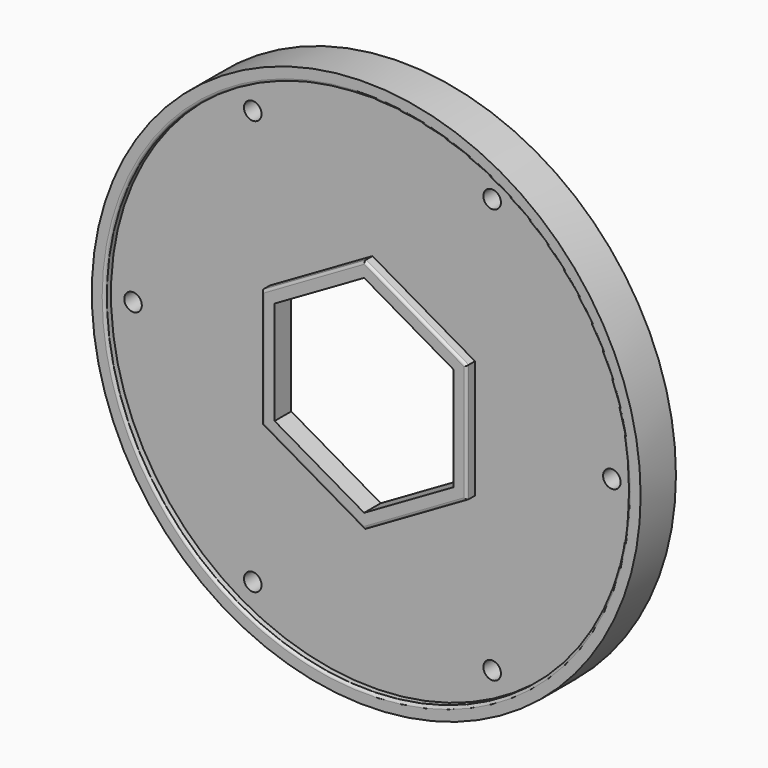
from build123d import *

# Parameters (mm, degrees)
F0_R          = 100.75
F0_R_2        = 5
F0_R_3        = 5.5430968475
F1_DEPTH      = 4
F2_DEPTH      = 4
F3_DEPTH      = 8
F0_R_4        = 105.75
F4_DEPTH      = 7
F6_R          = 1
F7_D          = 6.7564
F8_R          = 1
F9_DEPTH      = 7
F10_DEPTH     = 10
F11_D         = 6.7564
F12_R         = 1
F0_W          = 20
F0_H          = 5
F0_W_2        = 5
F0_H_2        = 20
F13_DEPTH     = 4
F14_DEPTH     = 12
F15_R         = 2
F16_T1_DEPTH  = 8
F16_T3_DEPTH  = 8
F16_T5_DEPTH  = 8
F16_T7_DEPTH  = 8
F16_S11_W     = 2
F16_S11_H     = 2
F16_T12_DEPTH = 2
F16_S17_W     = 2
F16_S17_H     = 2
F16_T18_DEPTH = 2
F16_S23_W     = 2
F16_S23_H     = 2
F16_T24_DEPTH = 2
F16_S29_W     = 2
F16_S29_H     = 2
F16_T30_DEPTH = 2
F16_S35_W     = 2
F16_S35_H     = 2
F16_T36_DEPTH = 2
F16_S41_W     = 2
F16_S41_H     = 2
F16_T42_DEPTH = 2
F16_S47_W     = 2
F16_S47_H     = 2
F16_T48_DEPTH = 2
F16_S53_W     = 2
F16_S53_H     = 2
F16_T54_DEPTH = 2


# Not quite as in the source:
# - a fillet or chamfer that OpenCascade refuses, or shapes differently, is made with other operations: its cross-section is extruded or revolved along the edge and cut away or added
# - a feature names something its author has since deleted; it is built from what else it names


with BuildPart() as f1:
    # F0 (on Front) → F1 (new body)
    with BuildSketch(Plane.XZ):
        Circle(F0_R)
        with Locations((-46.125, -79.8908434991)):
            Circle(F0_R_2, mode=Mode.SUBTRACT)
        with Locations((46.125, -79.8908434991)):
            Circle(F0_R_3, mode=Mode.SUBTRACT)
        with Locations((-92.25, 0)):
            Circle(F0_R_2, mode=Mode.SUBTRACT)
        with Locations((-46.125, 79.8908434991)):
            Circle(F0_R_2, mode=Mode.SUBTRACT)
        Polygon((80.5, 46.4766966698), (80.5, -46.4766966698), (0, -92.9533933395), (-80.5, -46.4766966698), (-80.5, 46.4766966698), (0, 92.9533933395), align=None, mode=Mode.SUBTRACT)
        with Locations((92.25, 0)):
            Circle(F0_R_2, mode=Mode.SUBTRACT)
        with Locations((46.125, 79.8908434991)):
            Circle(F0_R_2, mode=Mode.SUBTRACT)
        with Locations((46.125, 79.8908434991)):
            Circle(F0_R_2)
        with Locations((92.25, 0)):
            Circle(F0_R_2)
        with Locations((46.125, -79.8908434991)):
            Circle(F0_R_3)
        with Locations((-46.125, -79.8908434991)):
            Circle(F0_R_2)
        with Locations((-92.25, 0)):
            Circle(F0_R_2)
        with Locations((-46.125, 79.8908434991)):
            Circle(F0_R_2)
    extrude(amount=F1_DEPTH)



with BuildPart() as f1b:
    # F0 (on Front) → F1, piece 2 (new body)
    with BuildSketch(Plane.XZ):
        Polygon((77.5, -44.7446458622), (77.5, 44.7446458622), (0, 89.4892917244), (-77.5, 44.7446458622), (-77.5, -44.7446458622), (0, -89.4892917244), align=None)
        Polygon((49.9, -10), (49.9, -49.9), (10, -49.9), (10, -54.9), (-10, -54.9), (-10, -49.9), (-49.9, -49.9), (-49.9, -10), (-54.9, -10), (-54.9, 10), (-49.9, 10), (-49.9, 49.9), (-10, 49.9), (-10, 54.9), (10, 54.9), (10, 49.9), (49.9, 49.9), (49.9, 10), (54.9, 10), (54.9, -10), align=None, mode=Mode.SUBTRACT)
        Polygon((10, -49.9), (49.9, -49.9), (49.9, -10), (49.9, 10), (49.9, 49.9), (10, 49.9), (-10, 49.9), (-49.9, 49.9), (-49.9, 10), (-49.9, -10), (-49.9, -49.9), (-10, -49.9), align=None)
        Polygon((39.5, 22.805335633), (39.5, -22.805335633), (0, -45.610671266), (-39.5, -22.805335633), (-39.5, 22.805335633), (0, 45.610671266), align=None, mode=Mode.SUBTRACT)
    extrude(amount=F1_DEPTH)


with BuildPart() as f1_1:
    add(f1.part)

    add(f1b.part)  # F2 merges F1b
    # F0 (on Front) → F2 (join)
    with BuildSketch(Plane.XZ):
        Polygon((0, -92.9533933395), (80.5, -46.4766966698), (80.5, 46.4766966698), (0, 92.9533933395), (-80.5, 46.4766966698), (-80.5, -46.4766966698), align=None)
        Polygon((0, 89.4892917244), (77.5, 44.7446458622), (77.5, -44.7446458622), (0, -89.4892917244), (-77.5, -44.7446458622), (-77.5, 44.7446458622), align=None, mode=Mode.SUBTRACT)
    extrude(amount=F2_DEPTH)

    # F0 (on Front) → F3 (join)
    with BuildSketch(Plane.XZ):
        Polygon((0, -45.610671266), (39.5, -22.805335633), (39.5, 22.805335633), (0, 45.610671266), (-39.5, 22.805335633), (-39.5, -22.805335633), align=None)
        Polygon((34.5, 19.918584287), (34.5, -19.918584287), (0, -39.8371685741), (-34.5, -19.918584287), (-34.5, 19.918584287), (0, 39.8371685741), align=None, mode=Mode.SUBTRACT)
    extrude(amount=F3_DEPTH)

    # F0 (on Front) → F4 (join)
    with BuildSketch(Plane.XZ):
        Circle(F0_R_4)
        Circle(F0_R, mode=Mode.SUBTRACT)
    extrude(amount=F4_DEPTH)

    # F5: union 

    # F6
    f6_edges = [f1_1.edges().sort_by_distance(p)[0] for p in [
        (19.75, -8, 34.208003),
        (39.5, -8, 0),
        (19.75, -8, -34.208003),
        (-19.75, -8, -34.208003),
        (-39.5, -8, 0),
        (-19.75, -8, 34.208003),
    ]]
    fillet(f6_edges, radius=F6_R)

    # F7 (through all)
    with Locations(Plane(origin=(0, 0, 0), x_dir=(1, 0, 0), z_dir=(0, 1, 0))):
        with Locations((-46.125, -79.8908434991), (46.125, -79.8908434991), (92.25, 0), (46.125, 79.8908434991), (-46.125, 79.8908434991), (-92.25, 0)):
            Hole(F7_D / 2)

    # F8
    f8_edges = [f1_1.edges().sort_by_distance(p)[0] for p in [
        (-100.75, -7, 0),
    ]]
    fillet(f8_edges, radius=F8_R)

    # F0 (on Front) → F9 (join)
    with BuildSketch(Plane.XZ):
        with Locations((-46.125, 79.8908434991)):
            Circle(F0_R_2)
        with Locations((46.125, 79.8908434991)):
            Circle(F0_R_2)
        with Locations((92.25, 0)):
            Circle(F0_R_2)
        with Locations((46.125, -79.8908434991)):
            Circle(F0_R_3)
        with Locations((-46.125, -79.8908434991)):
            Circle(F0_R_2)
        with Locations((-92.25, 0)):
            Circle(F0_R_2)
    extrude(amount=-F9_DEPTH)

    # F0 (on Front) → F10 (join)
    with BuildSketch(Plane.XZ):
        Circle(F0_R_4)
        Circle(F0_R, mode=Mode.SUBTRACT)
    extrude(amount=-F10_DEPTH)

    # F11 (through all)
    with Locations(Plane.XZ):
        with Locations((-46.125, 79.8908434991), (46.125, 79.8908434991), (92.25, 0), (46.125, -79.8908434991), (-46.125, -79.8908434991), (-92.25, 0)):
            Hole(F11_D / 2)

    # F12
    f12_edges = [f1_1.edges().sort_by_distance(p)[0] for p in [
        (-100.75, 10, 0),
    ]]
    fillet(f12_edges, radius=F12_R)

    # F0 (on Front) → F13 (join)
    with BuildSketch(Plane.XZ):
        with Locations((0, -52.4)):
            Rectangle(F0_W, F0_H)
        with Locations((52.4, 0)):
            Rectangle(F0_W_2, F0_H_2)
        with Locations((0, 52.4)):
            Rectangle(F0_W, F0_H)
        with Locations((-52.4, 0)):
            Rectangle(F0_W_2, F0_H_2)
    extrude(amount=F13_DEPTH)

    # F0 (on Front) → F14 (join)
    with BuildSketch(Plane.XZ):
        with Locations((0, -52.4)):
            Rectangle(F0_W, F0_H)
        with Locations((52.4, 0)):
            Rectangle(F0_W_2, F0_H_2)
        with Locations((0, 52.4)):
            Rectangle(F0_W, F0_H)
        with Locations((-52.4, 0)):
            Rectangle(F0_W_2, F0_H_2)
    extrude(amount=-F14_DEPTH)

    # F15
    f15_edges = [f1_1.edges().sort_by_distance(p)[0] for p in [
        (0, 12, -49.9),
        (49.9, 12, 0),
        (0, 12, 49.9),
        (-49.9, 12, 0),
        (-10, 6, -49.9),
        (49.9, 6, 10),
        (49.9, 6, -10),
        (10, 6, -49.9),
        (-49.9, 6, -10),
        (-49.9, 6, 10),
        (-10, 6, 49.9),
        (10, 6, 49.9),
    ]]
    fillet(f15_edges, radius=F15_R)

    # F16: fillet of radius 2 on 8 edges, made by hand

    # F16_s2 → F16_t1 (cut)
    with BuildSketch(Plane.XY.offset(-59.9)):
        with BuildLine():
            ThreePointArc((-10, 10), (-9.4142135624, 11.4142135624), (-8, 12))
            Line((-8, 12), (-10, 12))
            Line((-10, 12), (-10, 10))
        make_face()
        with BuildLine():
            ThreePointArc((10, 10), (9.4142135624, 11.4142135624), (8, 12))
            Line((8, 12), (10, 12))
            Line((10, 12), (10, 10))
        make_face()
    extrude(amount=F16_T1_DEPTH, mode=Mode.SUBTRACT)

    # F16_s4 → F16_t3 (cut)
    with BuildSketch(Plane.YZ.offset(51.9)):
        with BuildLine():
            ThreePointArc((10, 10), (11.4142135624, 9.4142135624), (12, 8))
            Line((12, 8), (12, 10))
            Line((12, 10), (10, 10))
        make_face()
        with BuildLine():
            ThreePointArc((10, -10), (11.4142135624, -9.4142135624), (12, -8))
            Line((12, -8), (12, -10))
            Line((12, -10), (10, -10))
        make_face()
    extrude(amount=F16_T3_DEPTH, mode=Mode.SUBTRACT)

    # F16_s6 → F16_t5 (cut)
    with BuildSketch(Plane.XY.offset(51.9)):
        with BuildLine():
            ThreePointArc((10, 10), (9.4142135624, 11.4142135624), (8, 12))
            Line((8, 12), (10, 12))
            Line((10, 12), (10, 10))
        make_face()
        with BuildLine():
            ThreePointArc((-10, 10), (-9.4142135624, 11.4142135624), (-8, 12))
            Line((-8, 12), (-10, 12))
            Line((-10, 12), (-10, 10))
        make_face()
    extrude(amount=F16_T5_DEPTH, mode=Mode.SUBTRACT)

    # F16_s8 → F16_t7 (cut)
    with BuildSketch(Plane.YZ.offset(-59.9)):
        with BuildLine():
            ThreePointArc((10, 10), (11.4142135624, 9.4142135624), (12, 8))
            Line((12, 8), (12, 10))
            Line((12, 10), (10, 10))
        make_face()
        with BuildLine():
            ThreePointArc((10, -10), (11.4142135624, -9.4142135624), (12, -8))
            Line((12, -8), (12, -10))
            Line((12, -10), (10, -10))
        make_face()
    extrude(amount=F16_T7_DEPTH, mode=Mode.SUBTRACT)


with BuildPart() as f16_tool10:
    # F16_s11 → F16_t12 (new body)
    with BuildSketch(Plane.XY.offset(-8)):
        with Locations((-50.9, 11)):
            Rectangle(F16_S11_W, F16_S11_H)
    extrude(amount=-F16_T12_DEPTH)

    # F16_s13 → F16_t14 (revolve, cut)
    with BuildSketch(Plane(origin=(-51.9, 10, -8), x_dir=(-0.7071067812, -0.7071067812, 0), z_dir=(0.7071067812, -0.7071067812, 0))):
        with BuildLine():
            ThreePointArc((0, -2), (2, 0), (0, 2))
            Line((0, 2), (0, -2))
        make_face()
    revolve(axis=Axis((-51.9, 10, -8), (0, 0, -1)), mode=Mode.SUBTRACT)


with BuildPart() as f1_2:
    add(f1_1.part)

    # F16_t9: cut F16_tool10
    add(f16_tool10.part, mode=Mode.SUBTRACT)


with BuildPart() as f16_tool16:
    # F16_s17 → F16_t18 (new body)
    with BuildSketch(Plane.XY.offset(8)):
        with Locations((-50.9, 11)):
            Rectangle(F16_S17_W, F16_S17_H)
    extrude(amount=F16_T18_DEPTH)

    # F16_s19 → F16_t20 (revolve, cut)
    with BuildSketch(Plane(origin=(-51.9, 10, 8), x_dir=(-0.7071067812, -0.7071067812, 0), z_dir=(-0.7071067812, 0.7071067812, 0))):
        with BuildLine():
            ThreePointArc((0, -2), (2, 0), (0, 2))
            Line((0, 2), (0, -2))
        make_face()
    revolve(axis=Axis((-51.9, 10, 8), (0, 0, 1)), mode=Mode.SUBTRACT)


with BuildPart() as f1_3:
    add(f1_2.part)

    # F16_t15: cut F16_tool16
    add(f16_tool16.part, mode=Mode.SUBTRACT)


with BuildPart() as f16_tool22:
    # F16_s23 → F16_t24 (new body)
    with BuildSketch(Plane.YZ.offset(-8)):
        with Locations((11, 50.9)):
            Rectangle(F16_S23_W, F16_S23_H)
    extrude(amount=-F16_T24_DEPTH)

    # F16_s25 → F16_t26 (revolve, cut)
    with BuildSketch(Plane(origin=(-8, 10, 51.9), x_dir=(0, -0.7071067812, 0.7071067812), z_dir=(0, -0.7071067812, -0.7071067812))):
        with BuildLine():
            ThreePointArc((0, -2), (2, 0), (0, 2))
            Line((0, 2), (0, -2))
        make_face()
    revolve(axis=Axis((-8, 10, 51.9), (-1, 0, 0)), mode=Mode.SUBTRACT)


with BuildPart() as f1_4:
    add(f1_3.part)

    # F16_t21: cut F16_tool22
    add(f16_tool22.part, mode=Mode.SUBTRACT)


with BuildPart() as f16_tool28:
    # F16_s29 → F16_t30 (new body)
    with BuildSketch(Plane.YZ.offset(8)):
        with Locations((11, 50.9)):
            Rectangle(F16_S29_W, F16_S29_H)
    extrude(amount=F16_T30_DEPTH)

    # F16_s31 → F16_t32 (revolve, cut)
    with BuildSketch(Plane(origin=(8, 10, 51.9), x_dir=(0, -0.7071067812, 0.7071067812), z_dir=(0, 0.7071067812, 0.7071067812))):
        with BuildLine():
            ThreePointArc((0, -2), (2, 0), (0, 2))
            Line((0, 2), (0, -2))
        make_face()
    revolve(axis=Axis((8, 10, 51.9), (1, 0, 0)), mode=Mode.SUBTRACT)


with BuildPart() as f1_5:
    add(f1_4.part)

    # F16_t27: cut F16_tool28
    add(f16_tool28.part, mode=Mode.SUBTRACT)


with BuildPart() as f16_tool34:
    # F16_s35 → F16_t36 (new body)
    with BuildSketch(Plane.XY.offset(-8)):
        with Locations((50.9, 11)):
            Rectangle(F16_S35_W, F16_S35_H)
    extrude(amount=-F16_T36_DEPTH)

    # F16_s37 → F16_t38 (revolve, cut)
    with BuildSketch(Plane(origin=(51.9, 10, -8), x_dir=(0.7071067812, -0.7071067812, 0), z_dir=(0.7071067812, 0.7071067812, 0))):
        with BuildLine():
            ThreePointArc((0, -2), (2, 0), (0, 2))
            Line((0, 2), (0, -2))
        make_face()
    revolve(axis=Axis((51.9, 10, -8), (0, 0, -1)), mode=Mode.SUBTRACT)


with BuildPart() as f1_6:
    add(f1_5.part)

    # F16_t33: cut F16_tool34
    add(f16_tool34.part, mode=Mode.SUBTRACT)


with BuildPart() as f16_tool40:
    # F16_s41 → F16_t42 (new body)
    with BuildSketch(Plane.XY.offset(8)):
        with Locations((50.9, 11)):
            Rectangle(F16_S41_W, F16_S41_H)
    extrude(amount=F16_T42_DEPTH)

    # F16_s43 → F16_t44 (revolve, cut)
    with BuildSketch(Plane(origin=(51.9, 10, 8), x_dir=(0.7071067812, -0.7071067812, 0), z_dir=(-0.7071067812, -0.7071067812, 0))):
        with BuildLine():
            ThreePointArc((0, -2), (2, 0), (0, 2))
            Line((0, 2), (0, -2))
        make_face()
    revolve(axis=Axis((51.9, 10, 8), (0, 0, 1)), mode=Mode.SUBTRACT)


with BuildPart() as f1_7:
    add(f1_6.part)

    # F16_t39: cut F16_tool40
    add(f16_tool40.part, mode=Mode.SUBTRACT)


with BuildPart() as f16_tool46:
    # F16_s47 → F16_t48 (new body)
    with BuildSketch(Plane.YZ.offset(8)):
        with Locations((11, -50.9)):
            Rectangle(F16_S47_W, F16_S47_H)
    extrude(amount=F16_T48_DEPTH)

    # F16_s49 → F16_t50 (revolve, cut)
    with BuildSketch(Plane(origin=(8, 10, -51.9), x_dir=(0, -0.7071067812, -0.7071067812), z_dir=(0, -0.7071067812, 0.7071067812))):
        with BuildLine():
            ThreePointArc((0, -2), (2, 0), (0, 2))
            Line((0, 2), (0, -2))
        make_face()
    revolve(axis=Axis((8, 10, -51.9), (1, 0, 0)), mode=Mode.SUBTRACT)


with BuildPart() as f1_8:
    add(f1_7.part)

    # F16_t45: cut F16_tool46
    add(f16_tool46.part, mode=Mode.SUBTRACT)


with BuildPart() as f16_tool52:
    # F16_s53 → F16_t54 (new body)
    with BuildSketch(Plane.YZ.offset(-8)):
        with Locations((11, -50.9)):
            Rectangle(F16_S53_W, F16_S53_H)
    extrude(amount=-F16_T54_DEPTH)

    # F16_s55 → F16_t56 (revolve, cut)
    with BuildSketch(Plane(origin=(-8, 10, -51.9), x_dir=(0, -0.7071067812, -0.7071067812), z_dir=(0, 0.7071067812, -0.7071067812))):
        with BuildLine():
            ThreePointArc((0, -2), (2, 0), (0, 2))
            Line((0, 2), (0, -2))
        make_face()
    revolve(axis=Axis((-8, 10, -51.9), (-1, 0, 0)), mode=Mode.SUBTRACT)


with BuildPart() as f1_9:
    add(f1_8.part)

    # F16_t51: cut F16_tool52
    add(f16_tool52.part, mode=Mode.SUBTRACT)


solid = f1_9.part
